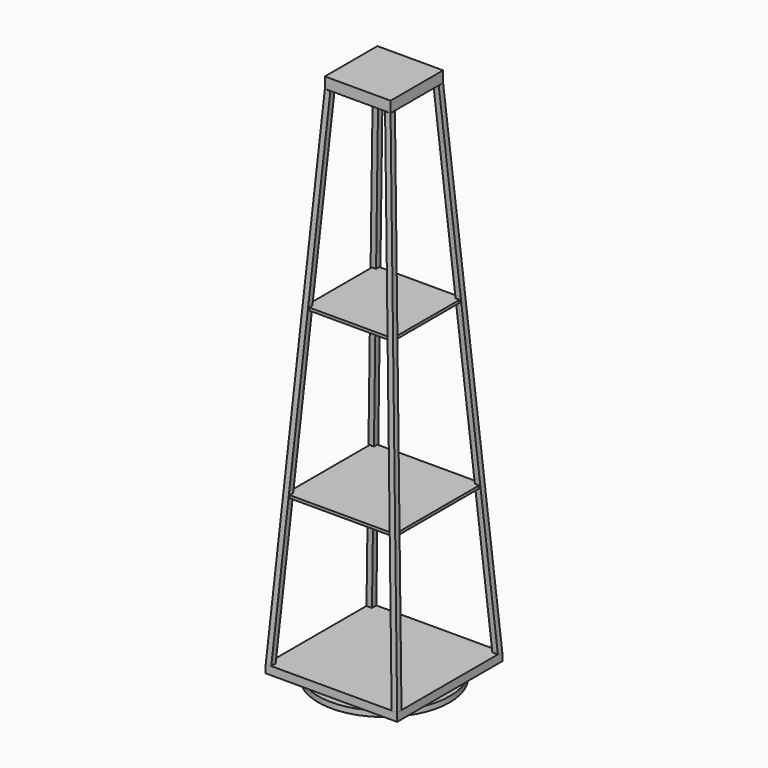
from build123d import *

# Parameters (mm, degrees)
F0_R      = 152.4
F1_DEPTH  = 12.7
F2_W      = 152.4
F2_H      = 152.4
F3_DEPTH  = 9.525
F4_W      = 304.8
F4_H      = 304.8
F5_DEPTH  = 19.05
F7_W      = 152.4
F7_H      = 152.4
F8_DEPTH  = 25.4
F11_DEPTH = 12.7
F13_W     = 254
F13_H     = 254
F14_DEPTH = 6.35
F16_W     = 203.2
F16_H     = 203.2
F17_DEPTH = 6.35


# Not quite as in the source:
# - a pattern or mirror of a feature is missing from the dataset's text; its kind, count and spacing are read off the source's solid


with BuildPart() as f1:
    # F0 (on Top) → F1 (new body)
    with BuildSketch(Plane.XY):
        Circle(F0_R)
    extrude(amount=F1_DEPTH)

    # F2 (on face) → F3 (join)
    with BuildSketch(Plane.XY.offset(12.7)):
        Rectangle(F2_W, F2_H)
    extrude(amount=F3_DEPTH)

    # F4 (on face) → F5 (join)
    with BuildSketch(Plane.XY.offset(22.225)):
        Rectangle(F4_W, F4_H)
    extrude(amount=F5_DEPTH)

    # F10 (on 3pt) → F11 (join)
    with BuildSketch(Plane(origin=(0, -154.4349882353, 10.0718470588), x_dir=(-1, 0, 0), z_dir=(0, 0.997880106, -0.0650791373))):
        Polygon((152.4, 31.2694408423), (76.2, 1202.1515869185), (63.5268089897, 1201.3268265801), (139.7268089897, 30.4446805039), align=None)
        Polygon((-63.5268089897, 1201.3268265801), (-76.2, 1202.1515869185), (-152.4, 31.2694408423), (-139.7268089897, 30.4446805039), align=None)
    f11 = extrude(amount=F11_DEPTH)

    # F11_copies: F11 across plane
    add(f11.mirror(Plane.ZX))

    # F13 (on offset) → F14 (join)
    with BuildSketch(Plane.XY.offset(381)):
        Rectangle(F13_W, F13_H)
    extrude(amount=F14_DEPTH)

    # F16 (on offset) → F17 (join)
    with BuildSketch(Plane.XY.offset(762)):
        Rectangle(F16_W, F16_H)
    extrude(amount=F17_DEPTH)


with BuildPart() as f8:
    # F7 (on offset) → F8 (new body)
    with BuildSketch(Plane.XY.offset(1209.675)):
        Rectangle(F7_W, F7_H)
    extrude(amount=F8_DEPTH)


solid = Compound([f1.part, f8.part])
